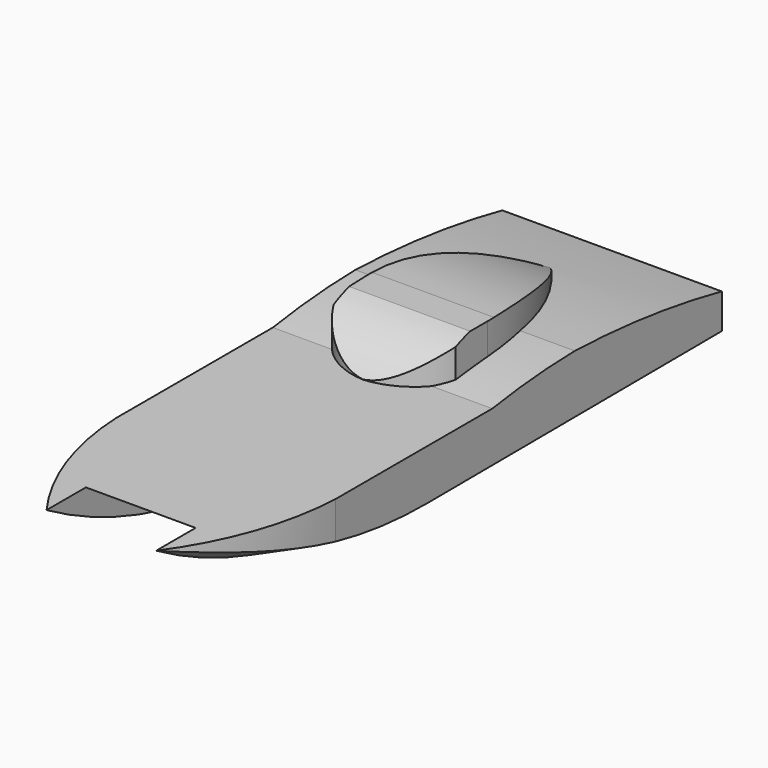
from build123d import *

# Parameters (mm, degrees)
F1_DEPTH  = 3352.8
F3_DEPTH  = 914.4
F5_DEPTH  = 3352.8
F7_W      = 1676.4
F7_H      = 187.770880038
F7_H_2    = 355.604804315
F10_DEPTH = 1320.8


with BuildPart() as f1:
    # F0 (on Right) → F1 (new body)
    with BuildSketch(Plane.YZ):
        with BuildLine():
            Line((9906.1763013826, 2286.2513795817), (9903.4036295408, 2819.6441732065))
            ThreePointArc((9903.4036295408, 2819.6441732065), (8507.7575621146, 3053.498500359), (7096.718104665, 3160.6593204871))
            ThreePointArc((7096.718104665, 3160.6593204871), (6306.1105449526, 3120.5478052313), (5520.2173816261, 3025.4626698664))
            Line((5520.2173816261, 3025.4626698664), (149.9354032589, 3025.4626698664))
            ThreePointArc((149.9354032589, 3025.4626698664), (2186.9166194611, 2445.3700036504), (4296.5021474202, 2257.0912826433))
            Line((4296.5021474202, 2257.0912826433), (9906.1763013826, 2286.2513795817))
        make_face()
        with BuildLine():
            Line((9906.1763013826, 1930.6465752666), (9906.1763013826, 2286.2513795817))
            Line((9906.1763013826, 2286.2513795817), (4296.5021474202, 2257.0912826433))
            ThreePointArc((4296.5021474202, 2257.0912826433), (2186.9166194611, 2445.3700036504), (149.9354032589, 3025.4626698664))
            ThreePointArc((149.9354032589, 3025.4626698664), (2147.8725687033, 2181.9750901472), (4298.3505953147, 1901.4960868935))
            Line((4298.3505953147, 1901.4960868935), (9906.1763013826, 1930.6465752666))
        make_face()
    extrude(amount=F1_DEPTH)

    # F2 (on face) → F3 (join)
    with BuildSketch(Plane.XY.offset(3025.4626698664)):
        with BuildLine():
            ThreePointArc((1683.8150913295, 5139.8680466252), (2221.5916744575, 5336.534299223), (2590.8, 5774.2173816261))
            Line((2590.8, 5774.2173816261), (2590.8, 6383.8173816261))
            ThreePointArc((2590.8, 6383.8173816261), (2336.9387512428, 7687.9813910632), (1612.4259228504, 8801.700592041))
            ThreePointArc((1612.4259228504, 8801.700592041), (931.872095069, 7660.5889477995), (729.0350215534, 6347.5213871845))
            Line((729.0350215534, 6347.5213871845), (752.7948753911, 5738.3845968446))
            ThreePointArc((752.7948753911, 5738.3845968446), (1138.7818511996, 5315.4244063088), (1683.8150913295, 5139.8680466252))
        make_face()
    extrude(amount=F3_DEPTH)

    # F4 (on face) → F5 (cut)
    with BuildSketch(Plane.YZ.offset(3352.8)):
        with BuildLine():
            ThreePointArc((5137.4154090881, 3025.4626698664), (5549.4088046364, 3384.9807891534), (6051.2724639455, 3602.0630397775))
            Line((6051.2724639455, 3602.0630397775), (6508.4724639455, 3602.0630397775))
            ThreePointArc((6508.4724639455, 3602.0630397775), (7699.4079318865, 3452.4470342276), (8816.3271482832, 3012.8976036053))
            Line((8816.3271482832, 3012.8976036053), (8976.5672683716, 4052.9136657715))
            Line((8976.5672683716, 4052.9136657715), (5137.4154090881, 4052.9136657715))
            Line((5137.4154090881, 4052.9136657715), (5137.4154090881, 3025.4626698664))
        make_face()
    extrude(amount=-F5_DEPTH, mode=Mode.SUBTRACT)

    # F8: sweep along a path in F8_path
    with BuildLine(Plane(origin=(3352.8, 9906.1763013826, 1930.6465752666), x_dir=(0, 0, 1), z_dir=(1, 0, 0))) as f8_path:
        Line((0, 0), (-29.1504883732, 5607.8257060679))
        ThreePointArc((-29.1504883732, 5607.8257060679), (251.3285148806, 7758.3037326792), (1094.8160945997, 9756.2408981237))
    # F7 (on face) → F8 (sweep, cut)
    with BuildSketch(Plane(origin=(0, 9906.1763013826, 0), x_dir=(-1, 0, 0), z_dir=(0, 1, 0))):
        Polygon((-2520.95, 1930.6465752666), (-3352.8, 2286.2513795817), (-3352.8, 1930.6465752666), align=None)
        Polygon((-2514.6, 1742.8756952286), (-2514.6, 1930.6465752666), (-2520.95, 1930.6465752666), (-3352.8, 1930.6465752666), (-3352.8, 1742.8756952286), align=None)
        with Locations((-1676.4, 1836.7611352476)):
            Rectangle(F7_W, F7_H)
        Polygon((-831.85, 1930.6465752666), (-838.2, 1930.6465752666), (-838.2, 1742.8756952286), (192.50908494, 1742.8756952286), (381.6066980362, 2006.4663887024), (0, 2286.2513795817), (0, 1930.6465752666), align=None)
        Polygon((0, 1930.6465752666), (0, 2286.2513795817), (-831.85, 1930.6465752666), align=None)
        with Locations((-1676.4, 2108.4489774241)):
            Rectangle(F7_W, F7_H_2)
    sweep(path=f8_path.line, mode=Mode.SUBTRACT)

    # F9 (on face) → F10 (cut)
    with BuildSketch(Plane.XY.offset(3025.4626698664)):
        with BuildLine():
            ThreePointArc((0, 2524.5586190393), (-4.7947551509, 2729.1455643262), (0, 2933.732509613))
            Line((0, 2933.732509613), (-833.7602615356, 377.7640759945))
            Line((-833.7602615356, 377.7640759945), (830.6194482815, 150.9683626398))
            add(Edge.make_bspline(
                [(0, 901.5324430601), (41.2990684914, 860.9735825536), (82.7531470768, 820.7592729572), (124.3534648361, 780.8755615368), (166.0922333943, 741.3097367391), (249.3112654144, 663.2792388889), (290.7882589994, 624.8070025808), (332.386779466, 586.6219277036), (374.1008263909, 548.7136108018), (457.311819666, 473.8247323565), (498.8064651623, 436.8386233615), (540.4037012367, 400.1046584982), (582.0988058574, 363.6142038331), (665.0600262184, 291.6387661512), (706.3233958068, 256.1468967875), (747.673514319, 220.8758836415), (789.1066626784, 185.818597837), (830.6194482815, 150.9683626398)],
                knots=[0, 0, 0, 0, 0, 0, 0.2542407325, 0.2542407325, 0.2542407325, 0.2542407325, 0.505314854, 0.505314854, 0.505314854, 0.505314854, 0.7537635021, 0.7537635021, 0.7537635021, 0.7537635021, 0.9985488127, 0.9985488127, 0.9985488127, 0.9985488127, 0.9985488127, 0.9985488127], degree=5))
            Line((0, 901.5324430598), (0, 2524.5586190393))
        make_face()
        with BuildLine():
            ThreePointArc((838.2, 149.9354032589), (244.2280510065, 1275.5203057617), (0, 2524.5586190393))
            Line((0, 2524.5586190393), (0, 901.5324430598))
            add(Edge.make_bspline(
                [(0, 901.5324430601), (41.2990684914, 860.9735825536), (82.7531470768, 820.7592729572), (124.3534648361, 780.8755615368), (166.0922333943, 741.3097367391), (249.3112654144, 663.2792388889), (290.7882589994, 624.8070025808), (332.386779466, 586.6219277036), (374.1008263909, 548.7136108018), (457.311819666, 473.8247323565), (498.8064651623, 436.8386233615), (540.4037012367, 400.1046584982), (582.0988058574, 363.6142038331), (665.0600262184, 291.6387661512), (706.3233958068, 256.1468967875), (747.673514319, 220.8758836415), (789.1066626784, 185.818597837), (830.6194482815, 150.9683626398)],
                knots=[0, 0, 0, 0, 0, 0, 0.2542407325, 0.2542407325, 0.2542407325, 0.2542407325, 0.505314854, 0.505314854, 0.505314854, 0.505314854, 0.7537635021, 0.7537635021, 0.7537635021, 0.7537635021, 0.9985488127, 0.9985488127, 0.9985488127, 0.9985488127, 0.9985488127, 0.9985488127], degree=5))
            Line((830.6194482815, 150.9683626398), (838.2, 149.9354032589))
        make_face()
        with BuildLine():
            ThreePointArc((3352.8, 2524.5586190392), (3108.5719489935, 1275.5203057617), (2514.6, 149.9354032589))
            Line((2514.6, 149.9354032589), (2520.95, 149.9354032589))
            add(Edge.make_bspline(
                [(2520.95, 149.9354032589), (2562.7107893152, 184.9873072693), (2604.3910553646, 220.248604014), (2645.9873487862, 255.7260842272), (2687.4958862315, 291.4270008447), (2770.7011941431, 363.6142038335), (2812.3962987638, 400.1046584985), (2853.9935348381, 436.8386233618), (2895.4881803343, 473.8247323568), (2978.6991736092, 548.7136108019), (3020.4132205339, 586.6219277035), (3062.0117410005, 624.8070025807), (3103.4887345854, 663.2792388887), (3186.7077666055, 741.3097367389), (3228.4465351637, 780.8755615366), (3270.0468529231, 820.7592729571), (3311.5009315086, 860.9735825535), (3352.8, 901.5324430601)],
                knots=[0, 0, 0, 0, 0, 0, 0.2462364979, 0.2462364979, 0.2462364979, 0.2462364979, 0.494685146, 0.494685146, 0.494685146, 0.494685146, 0.7457592675, 0.7457592675, 0.7457592675, 0.7457592675, 1, 1, 1, 1, 1, 1], degree=5))
            Line((3352.8, 901.5324430598), (3352.8, 2524.5586190392))
        make_face()
        with BuildLine():
            ThreePointArc((3352.8, 2933.732509613), (3357.5947551509, 2729.1455643261), (3352.8, 2524.5586190392))
            Line((3352.8, 2524.5586190392), (3352.8, 901.5324430598))
            add(Edge.make_bspline(
                [(2520.95, 149.9354032589), (2562.7107893152, 184.9873072693), (2604.3910553646, 220.248604014), (2645.9873487862, 255.7260842272), (2687.4958862315, 291.4270008447), (2770.7011941431, 363.6142038335), (2812.3962987638, 400.1046584985), (2853.9935348381, 436.8386233618), (2895.4881803343, 473.8247323568), (2978.6991736092, 548.7136108019), (3020.4132205339, 586.6219277035), (3062.0117410005, 624.8070025807), (3103.4887345854, 663.2792388887), (3186.7077666055, 741.3097367389), (3228.4465351637, 780.8755615366), (3270.0468529231, 820.7592729571), (3311.5009315086, 860.9735825535), (3352.8, 901.5324430601)],
                knots=[0, 0, 0, 0, 0, 0, 0.2462364979, 0.2462364979, 0.2462364979, 0.2462364979, 0.494685146, 0.494685146, 0.494685146, 0.494685146, 0.7457592675, 0.7457592675, 0.7457592675, 0.7457592675, 1, 1, 1, 1, 1, 1], degree=5))
            Line((2520.95, 149.9354032589), (4820.351600647, 149.9354032589))
            Line((4820.351600647, 149.9354032589), (3352.8, 2933.732509613))
        make_face()
    extrude(amount=-F10_DEPTH, mode=Mode.SUBTRACT)


solid = f1.part
